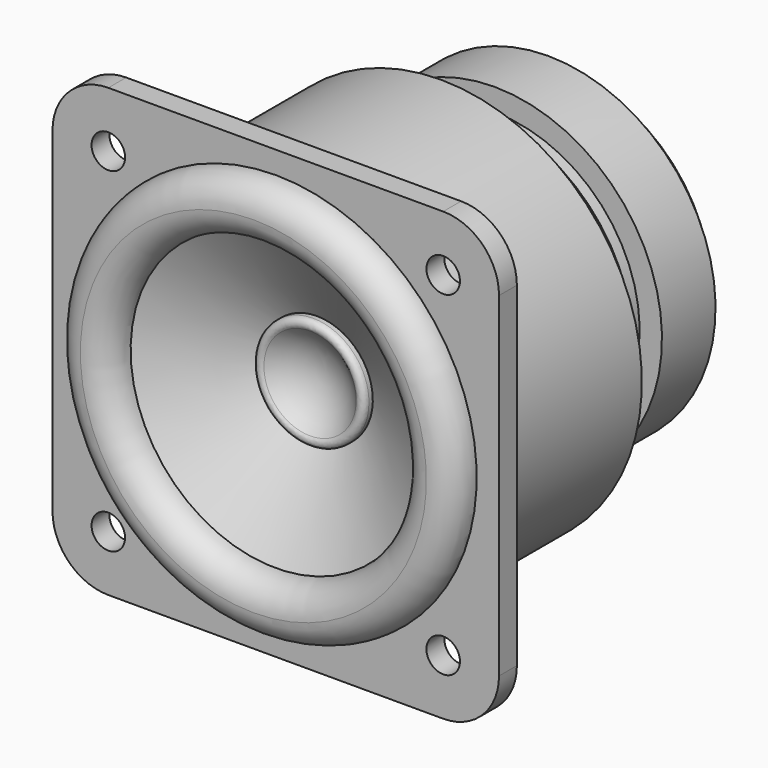
from build123d import *

# Parameters (mm, degrees)
F0_W             = 40
F0_H             = 40
F1_DEPTH         = 2
F2_R             = 5
F3_R             = 18
F4_DEPTH         = 2
F7_R             = 2.49999
F8_R             = 0.5
F10_D            = 3
F10_COPIES_COUNT = 4


# Not quite as in the source:
# - a fillet or chamfer is up to 0.001 mm smaller than in the source, because OpenCascade refuses the exact size
# - a pattern or mirror of a feature is missing from the dataset's text; its kind, count and spacing are read off the source's solid


with BuildPart() as f1:
    # F0 (on Front) → F1 (new body)
    with BuildSketch(Plane.XZ):
        Rectangle(F0_W, F0_H)
    extrude(amount=-F1_DEPTH)

    # F2
    f2_edges = [f1.edges().sort_by_distance(p)[0] for p in [
        (20, 1, 20),
        (20, 1, -20),
        (-20, 1, -20),
        (-20, 1, 20),
    ]]
    fillet(f2_edges, radius=F2_R)

    # F3 (on face) → F4 (cut, through all)
    with BuildSketch(Plane.XZ):
        Circle(F3_R)
    extrude(amount=-F4_DEPTH, mode=Mode.SUBTRACT)

    # F5 (on Right) → F6 (revolve)
    with BuildSketch(Plane.YZ):
        with BuildLine():
            Line((18.5, 18), (0, 18))
            Line((0, 18), (-2.5, 18))
            Line((-2.5, 18), (-2.5, 13))
            Line((-2.5, 13), (0, 13))
            Line((0, 13), (4.6188021535, 5))
            Line((4.6188021535, 5), (2.6188021535, 5))
            ThreePointArc((2.6188021535, 5), (4.8290490902, 2.9220557153), (5.6443001975, 0))
            Line((5.6443001975, 0), (32.5, 0))
            Line((32.5, 0), (32.5, 13))
            Line((32.5, 13), (30.5, 13))
            Line((30.5, 13), (30.5, 15))
            Line((30.5, 15), (24.5, 15))
            Line((24.5, 15), (24.5, 13))
            Line((24.5, 13), (22.5, 13))
            Line((22.5, 13), (22.5, 14))
            Line((22.5, 14), (21.5, 14))
            Line((21.5, 14), (21.5, 15))
            Line((21.5, 15), (19.5, 15))
            Line((19.5, 15), (19.5, 14))
            Line((19.5, 14), (18.5, 14))
            Line((18.5, 14), (18.5, 18))
        make_face()
    revolve(axis=Axis((0, 19.0721500987, 0), (0, -1, 0)))

    # F7 (radius 2.5 in the source; OpenCascade refuses exactly that, so slightly less here)
    f7_edges = [f1.edges().sort_by_distance(p)[0] for p in [
        (0, -2.5, -18),
        (0, -2.5, -13),
    ]]
    fillet(f7_edges, radius=F7_R)

    # F8
    f8_edges = [f1.edges().sort_by_distance(p)[0] for p in [
        (0, 2.618802, -5),
    ]]
    fillet(f8_edges, radius=F8_R)

    # F10 (through all)
    with Locations(Plane.XZ):
        with Locations((-15, 15)):
            f10 = Hole(F10_D / 2)

    # F10_copies: F10 ×4 about axis
    f10_copies_axis = Axis((0, 0, 0), (0, 1, 0))
    for i in range(1, F10_COPIES_COUNT):
        add(f10.rotate(f10_copies_axis, i * 360 / F10_COPIES_COUNT), mode=Mode.SUBTRACT)


solid = f1.part
